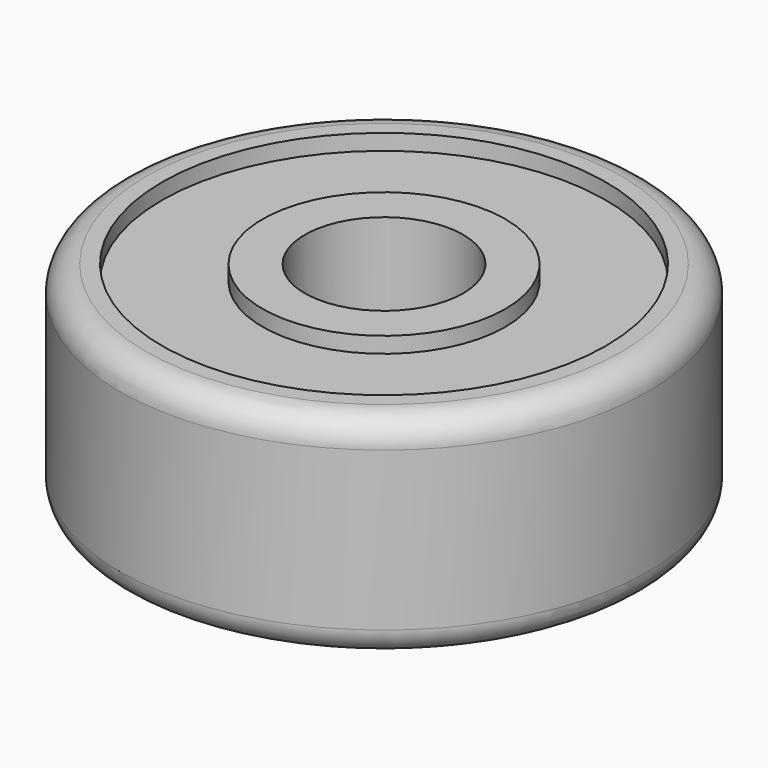
from build123d import *

# Parameters (mm, degrees)
F0_R     = 5
F0_R_2   = 4.2
F1_DEPTH = 3.5
F0_R_3   = 2.3
F2_DEPTH = 3.2
F0_R_4   = 1.5
F3_DEPTH = 3.5
F4_DEPTH = 0.5
F5_DEPTH = 0.5
F6_DEPTH = 0.2
F7_R     = 0.49999


# Not quite as in the source:
# - a fillet or chamfer is up to 0.001 mm smaller than in the source, because OpenCascade refuses the exact size


with BuildPart() as f1:
    # F0 (on Top) → F1 (new body)
    with BuildSketch(Plane.XY):
        Circle(F0_R)
        Circle(F0_R_2, mode=Mode.SUBTRACT)
    extrude(amount=F1_DEPTH)

    # F0 (on Top) → F2 (join)
    with BuildSketch(Plane.XY):
        Circle(F0_R_2)
        Circle(F0_R_3, mode=Mode.SUBTRACT)
    extrude(amount=F2_DEPTH)

    # F0 (on Top) → F3 (join)
    with BuildSketch(Plane.XY):
        Circle(F0_R_3)
        Circle(F0_R_4, mode=Mode.SUBTRACT)
    extrude(amount=F3_DEPTH)

    # F0 (on Top) → F4 (join)
    with BuildSketch(Plane.XY):
        Circle(F0_R)
        Circle(F0_R_2, mode=Mode.SUBTRACT)
    extrude(amount=-F4_DEPTH)

    # F0 (on Top) → F5 (join)
    with BuildSketch(Plane.XY):
        Circle(F0_R_3)
        Circle(F0_R_4, mode=Mode.SUBTRACT)
    extrude(amount=-F5_DEPTH)

    # F0 (on Top) → F6 (join)
    with BuildSketch(Plane.XY):
        Circle(F0_R_2)
        Circle(F0_R_3, mode=Mode.SUBTRACT)
    extrude(amount=-F6_DEPTH)

    # F7 (radius 0.5 in the source; OpenCascade refuses exactly that, so slightly less here)
    f7_edges = [f1.edges().sort_by_distance(p)[0] for p in [
        (-5, 0, 3.5),
        (-5, 0, -0.5),
    ]]
    fillet(f7_edges, radius=F7_R)


solid = f1.part
